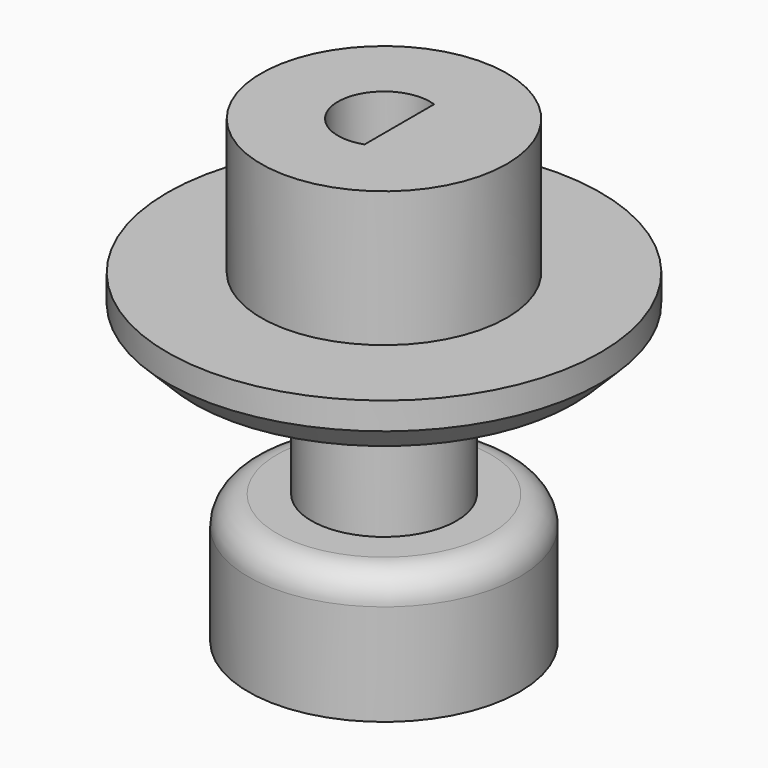
from build123d import *

# Parameters (mm, degrees)
F0_R      = 6.3637373436
F1_DEPTH  = 6.096
F2_R      = 3.4022099148
F3_DEPTH  = 12.7
F5_R      = 10.1544070979
F6_DEPTH  = 2.54
F8_R      = 5.7592976
F9_DEPTH  = 6.35
F12_DEPTH = 6.35
F13_D     = 10.16
F13_DEPTH = 1.27
F13_TIP   = 3.0523719447
F14_R     = 1.3490625387
F15_SIZE  = 1.27


with BuildPart() as f1:
    # F0 (on Top) → F1 (new body)
    with BuildSketch(Plane.XY):
        Circle(F0_R)
    extrude(amount=F1_DEPTH)

    # F2 (on Top) → F3 (join)
    with BuildSketch(Plane.XY):
        Circle(F2_R)
    extrude(amount=F3_DEPTH)

    # F5 (on offset) → F6 (join)
    with BuildSketch(Plane.XY.offset(12.7)):
        Circle(F5_R)
    extrude(amount=F6_DEPTH)

    # F8 (on offset) → F9 (join)
    with BuildSketch(Plane.XY.offset(15.24)):
        Circle(F8_R)
    extrude(amount=F9_DEPTH)

    # F11 (on offset) → F12 (cut)
    with BuildSketch(Plane.XY.offset(21.59)):
        with BuildLine():
            Line((0.7198907698, 0), (0.7198907698, 2.0371562))
            ThreePointArc((0.7198907698, 2.0371562), (-2.1606129, 0), (0.7198907698, -2.0371562))
            Line((0.7198907698, -2.0371562), (0.7198907698, 0))
        make_face()
    extrude(amount=-F12_DEPTH, mode=Mode.SUBTRACT)

    # F13
    with Locations(Plane(origin=(0, 0, 0), x_dir=(1, 0, 0), z_dir=(0, 0, -1))):
        with Locations((0, 0)):
            Hole(F13_D / 2, depth=F13_DEPTH)
            with Locations((0, 0, -(F13_DEPTH + F13_TIP / 2))):  # 118° drill point
                Cone(0, F13_D / 2, F13_TIP, mode=Mode.SUBTRACT)

    # F14
    f14_edges = [f1.edges().sort_by_distance(p)[0] for p in [
        (-6.363737, 0, 6.096),
    ]]
    fillet(f14_edges, radius=F14_R)

    # F15
    f15_edges = [f1.edges().sort_by_distance(p)[0] for p in [
        (-10.154407, 0, 12.7),
    ]]
    chamfer(f15_edges, length=F15_SIZE)


solid = f1.part
